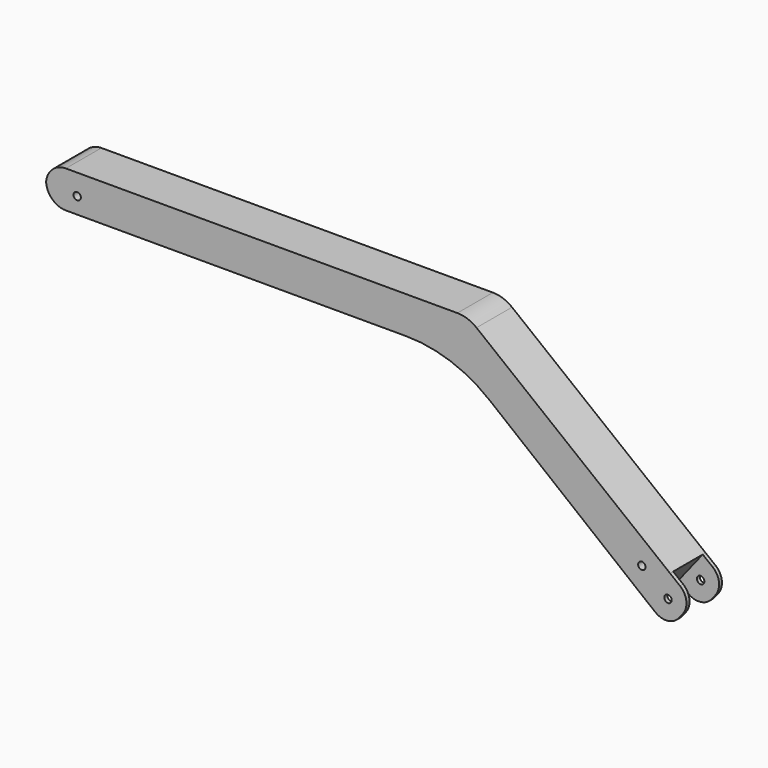
from build123d import *

# Parameters (mm, degrees)
F0_R        = 10
F1_DEPTH    = 120
F2_T1_DEPTH = 388.0868278764
F3_R        = 83.3946881549
F4_R        = 360.5996262689
F5_W        = 10.426518289
F5_H        = 107.3879271778
F5_W_2      = 9.573481711
F6_DEPTH    = 80
F7_T1_DEPTH = 238.837194796
F7_T3_DEPTH = 237.984158218
F9_D        = 20


# Not quite as in the source:
# - a fillet or chamfer that OpenCascade refuses, or shapes differently, is made with other operations: its cross-section is extruded or revolved along the edge and cut away or added


with BuildPart() as f1:
    # F0 (on Front) → F1 (new body)
    with BuildSketch(Plane.XZ):
        Polygon((240.6433847223, 159.6522270207), (-900.6182220181, 159.6522270207), (-900.6182220181, 59.6522270207), (200.0234600665, 59.6522270207), align=None)
        with Locations((-816.3304328918, 103.5160794854)):
            Circle(F0_R, mode=Mode.SUBTRACT)
        Polygon((786.7558863362, -272.8294734313), (240.6433847223, 159.6522270207), (200.0234600665, 59.6522270207), (720.0863678131, -357.0158274528), align=None)
        with Locations((710.3598117828, -279.6283066273)):
            Circle(F0_R, mode=Mode.SUBTRACT)
    extrude(amount=F1_DEPTH)

    # F2: fillet of radius 53.6173655753 on 2 edges, made by hand

    # F2_s2 → F2_t1 (cut)
    with BuildSketch(Plane.XZ.offset(-134.0434139382)):
        with BuildLine():
            ThreePointArc((-847.0008564428, 159.6522270207), (-884.9140592305, 143.9480642331), (-900.6182220181, 106.0348614454))
            Line((-900.6182220181, 106.0348614454), (-900.6182220181, 159.6522270207))
            Line((-900.6182220181, 159.6522270207), (-847.0008564428, 159.6522270207))
        make_face()
        with BuildLine():
            ThreePointArc((-900.6182220181, 113.269592596), (-884.9140592305, 75.3563898084), (-847.0008564428, 59.6522270207))
            Line((-847.0008564428, 59.6522270207), (-900.6182220181, 59.6522270207))
            Line((-900.6182220181, 59.6522270207), (-900.6182220181, 113.269592596))
        make_face()
    extrude(amount=F2_T1_DEPTH, mode=Mode.SUBTRACT)

    # F3
    f3_edges = [f1.edges().sort_by_distance(p)[0] for p in [
        (240.643385, -60, 159.652227),
    ]]
    fillet(f3_edges, radius=F3_R)

    # F4
    f4_edges = [f1.edges().sort_by_distance(p)[0] for p in [
        (200.02346, -60, 59.652227),
    ]]
    fillet(f4_edges, radius=F4_R)

    # F5 (on face) → F6 (join)
    with BuildSketch(Plane(origin=(616.3029320724, 0, -488.0674572886), x_dir=(0, 1, 0), z_dir=(0.7839461682, 0, -0.6208288052))):
        with Locations((-114.7867408555, 220.8631330454)):
            Rectangle(F5_W, F5_H)
        with Locations((-4.7867408555, 220.8631330454)):
            Rectangle(F5_W_2, F5_H)
    extrude(amount=F6_DEPTH)

    # F7: fillet of radius 45.6821353014 on 5 edges, made by hand

    # F7_s2 → F7_t1 (cut)
    with BuildSketch(Plane.XZ.offset(-4.6318565425)):
        with BuildLine():
            ThreePointArc((811.1628467471, -370.8697969446), (780.6195529663, -387.886260073), (746.9897263442, -378.3213463908))
            Line((746.9897263442, -378.3213463908), (782.8020612687, -406.6821318691))
            Line((782.8020612687, -406.6821318691), (811.1628467471, -370.8697969446))
        make_face()
        with BuildLine():
            ThreePointArc((821.1107943135, -358.3081127721), (830.6757079957, -324.6782861501), (813.6592448673, -294.1349923693))
            Line((813.6592448673, -294.1349923693), (849.4715797918, -322.4957778476))
            Line((849.4715797918, -322.4957778476), (821.1107943135, -358.3081127721))
        make_face()
    extrude(amount=F7_T1_DEPTH, mode=Mode.SUBTRACT)

    # F7_s4 → F7_t3 (cut)
    with BuildSketch(Plane.XZ.offset(-114.2053382535)):
        with BuildLine():
            ThreePointArc((811.1628467471, -370.8697969446), (780.6195529663, -387.886260073), (746.9897263442, -378.3213463908))
            Line((746.9897263442, -378.3213463908), (782.8020612687, -406.6821318691))
            Line((782.8020612687, -406.6821318691), (811.1628467471, -370.8697969446))
        make_face()
        with BuildLine():
            ThreePointArc((813.6592448673, -294.1349923693), (830.6757079957, -324.6782861501), (821.1107943135, -358.3081127721))
            Line((821.1107943135, -358.3081127721), (849.4715797918, -322.4957778476))
            Line((849.4715797918, -322.4957778476), (813.6592448673, -294.1349923693))
        make_face()
    extrude(amount=F7_T3_DEPTH, mode=Mode.SUBTRACT)

    # F9 (through all)
    with Locations(Plane(origin=(0, 0, 0), x_dir=(-1, 0, 0), z_dir=(0, 1, 0))):
        with Locations((-781.1415195465, -335.5341851711)):
            Hole(F9_D / 2)


solid = f1.part
